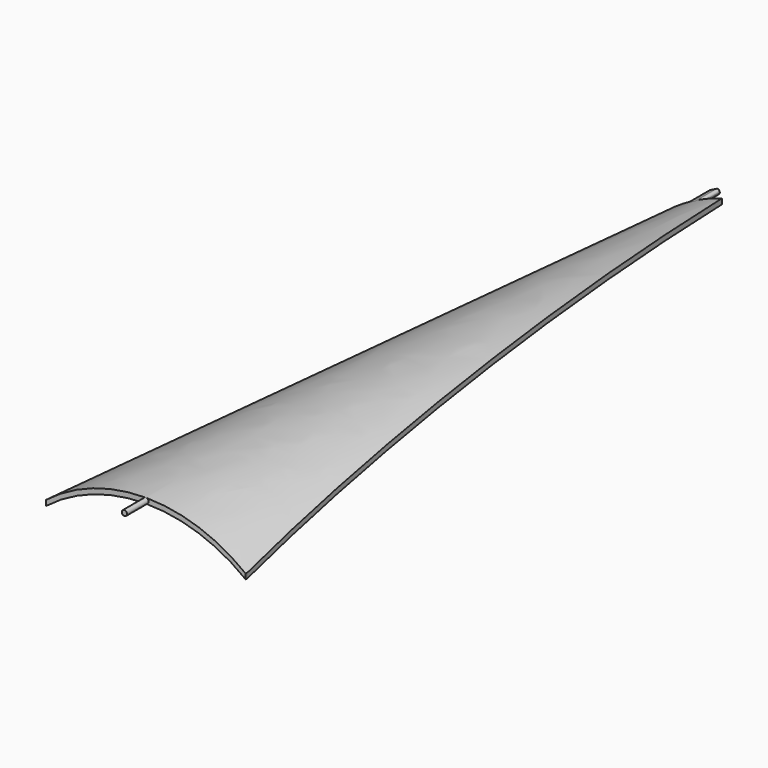
from build123d import *

# Parameters (mm, degrees)
F1_DEPTH = 25
F4_DEPTH = 10
F5_R     = 0.8
F6_R     = 0.9825772789
F7_DEPTH = 10


with BuildPart() as f1:
    # F0 (on Top) → F1 (new body)
    with BuildSketch(Plane.XY):
        Polygon((-37, -56.6475350804), (-2, -56.6475350804), (2, -56.6475350804), (37, -56.6475350804), (10, 197.3524649196), (2, 197.3524649196), (2, 196.3524649196), (-2, 196.3524649196), (-2, 197.3524649196), (-10, 197.3524649196), align=None)
    extrude(amount=F1_DEPTH)

    # F3: sweep along a path in F3_path
    with BuildLine(Plane(origin=(-10, 197.3524649196, 0), x_dir=(0.1057036895, 0.994397672, 0), z_dir=(-0.994397672, 0.1057036895, 0))) as f3_path:
        Line((0, 0), (-255.4310082977, 0))
    # F2 (on face) → F3 (sweep, intersect)
    with BuildSketch(Plane.XZ.offset(56.6475350804)):
        with BuildLine():
            ThreePointArc((-37, 0), (-0.0846525336, 12.7664775684), (36.8665717542, 0.1042166445))
            Line((36.8665717542, 0.1042166445), (36.8665717542, 2))
            ThreePointArc((36.8665717542, 2), (-0.0667141229, 14.7143531892), (-37, 2))
            Line((-37, 2), (-37, 0))
        make_face()
    sweep(path=f3_path.line, mode=Mode.INTERSECT)

    # F4 (add): a face of the model
    f4_faces = [f1.faces().sort_by_distance(p)[0] for p in [
        (-0.0010475513, 196.3524649196, 7.3762184587),
    ]]
    extrude(f4_faces, amount=F4_DEPTH)

    # F5
    f5_edges = [f1.edges().sort_by_distance(p)[0] for p in [
        (2, 201.852465, 7.358695),
        (2, 201.352465, 9.336883),
        (-2, 201.852465, 5.351269),
        (-2, 201.352465, 7.335688),
    ]]
    fillet(f5_edges, radius=F5_R)

    # F6 (on face) → F7 (join)
    with BuildSketch(Plane.XZ.offset(56.6475350804)):
        with Locations((0, 13.7826548889)):
            Circle(F6_R)
    extrude(amount=F7_DEPTH)


solid = f1.part
